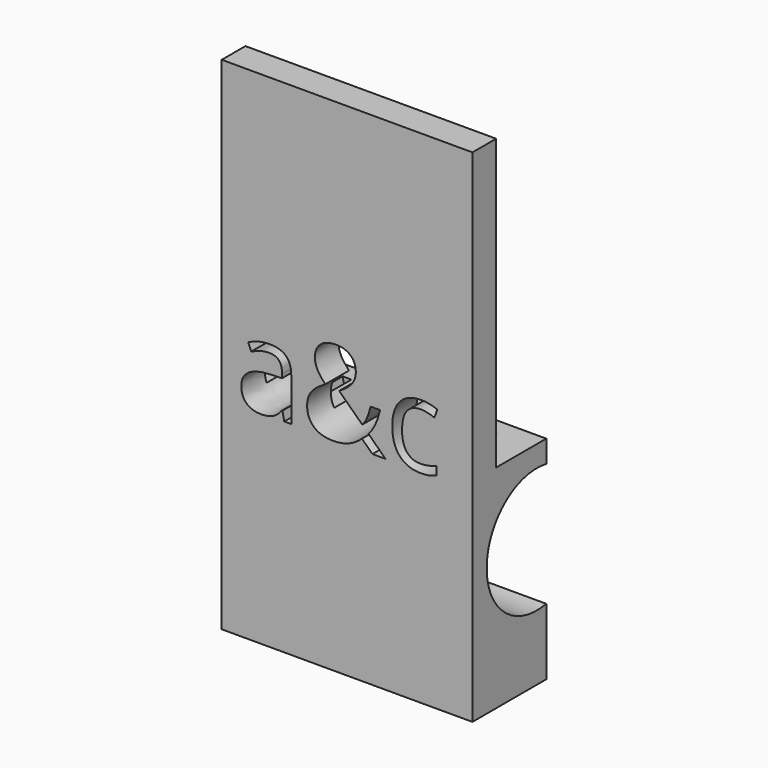
from build123d import *

# Parameters (mm, degrees)
F0_W         = 50.8
F0_H         = 101.6
F1_DEPTH     = 6
F2_R         = 2.5
F3_DEPTH     = 50.801
F4_TEXT_SIZE = 23.5962784953
F5_DEPTH     = 2.54
F7_DEPTH     = 12.7
F6_W         = 50.8
F6_H         = 58.6639862616
F8_DEPTH     = 12.7
F9_R         = 12.7
F10_DEPTH    = 50.8010001


# Not quite as in the source:
# - Text() gives the source's letters only with a copy of the font that has no kerning and outlines rounded to 1/6400 em; it was checked with that copy


with BuildPart() as f1:
    # F0 (on Front) → F1 (new body)
    with BuildSketch(Plane.XZ):
        with Locations((-25.4, 53.057777651)):
            Rectangle(F0_W, F0_H)
    extrude(amount=F1_DEPTH)

    # F2 (on face) → F3 (cut, through all)
    with BuildSketch(Plane.YZ):
        with Locations((-2.6137421373, 95.9439501166)):
            Circle(F2_R)
    extrude(amount=-F3_DEPTH, mode=Mode.SUBTRACT)

    # F4 (on face) → F5 (cut)
    with BuildSketch(Plane.XZ.offset(6)):
        with Locations((-47.9186000302, 43.4513017535)):
            Text('a&c', F4_TEXT_SIZE, font='Open Sans', text_align=(TextAlign.LEFT, TextAlign.BOTTOM))
    extrude(amount=-F5_DEPTH, mode=Mode.SUBTRACT)

    # F7 (add): a face of the model
    f7_faces = [f1.faces().sort_by_distance(p)[0] for p in [
        (-25.1754586765, -6, 53.2338693362),
    ]]
    extrude(f7_faces, amount=F7_DEPTH)

    # F6 (on face) → F8 (cut)
    with BuildSketch(Plane(origin=(0, 0, 0), x_dir=(-1, 0, 0), z_dir=(0, 1, 0))):
        with Locations((25.4, 74.5257845203)):
            Rectangle(F6_W, F6_H)
    extrude(amount=-F8_DEPTH, mode=Mode.SUBTRACT)

    # F9 (on face) → F10 (cut, through all)
    with BuildSketch(Plane.YZ):
        with Locations((-2.3959300015, 28.2044690102)):
            Circle(F9_R)
    extrude(amount=-F10_DEPTH, mode=Mode.SUBTRACT)


solid = f1.part
